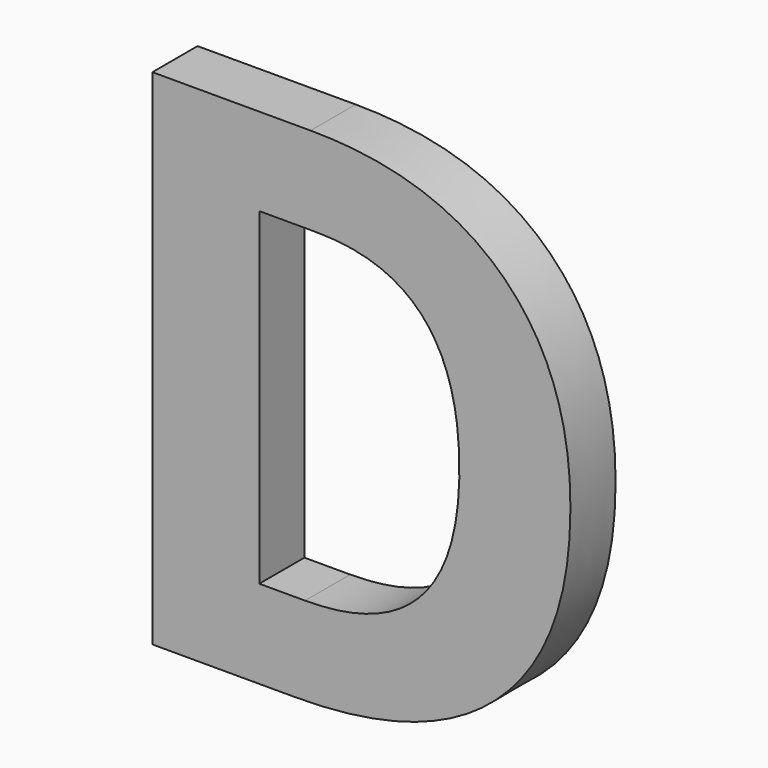
from build123d import *

# Parameters (mm, degrees)
F0_TEXT_SIZE = 62.5
F1_DEPTH     = 5


# Not quite as in the source:
# - Text() gives the source's letters only with a copy of the font that has no kerning and outlines rounded to 1/6400 em; it was checked with that copy


with BuildPart() as f1:
    # F0 (on Front) → F1 (new body)
    with BuildSketch(Plane.XZ):
        with Locations((-70.0147059366, 14.9558821901)):
            Text('D', F0_TEXT_SIZE, font='Open Sans', font_style=FontStyle.BOLD, text_align=(TextAlign.LEFT, TextAlign.BOTTOM))
    extrude(amount=F1_DEPTH)


solid = f1.part
